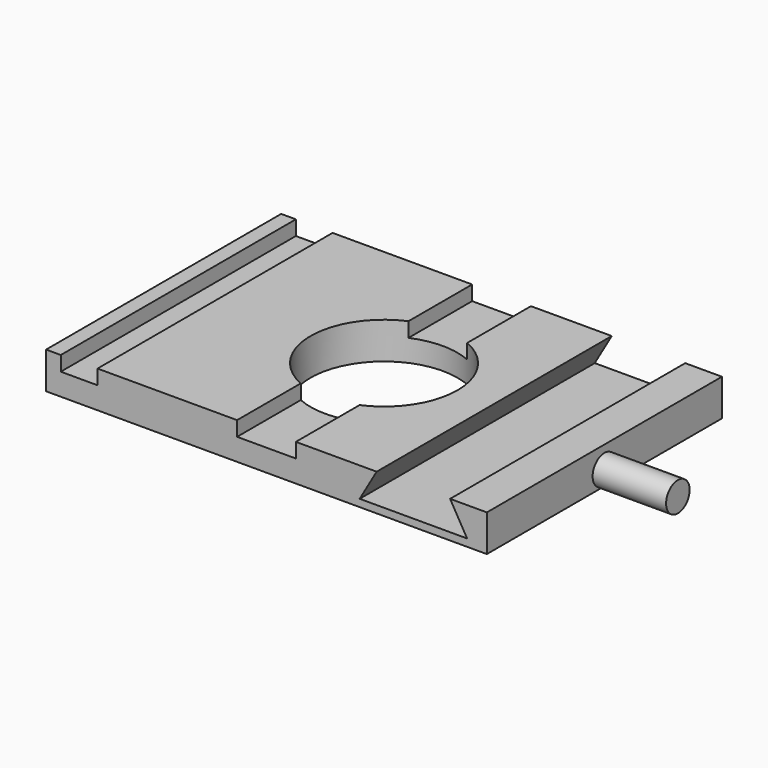
from build123d import *

# Parameters (mm, degrees)
F0_W     = 76.2
F0_H     = 50.8
F0_R     = 12.7
F1_DEPTH = 6.35
F2_W     = 6.35
F2_H     = 50.8
F3_DEPTH = 2.54
F5_DEPTH = 25.4
F6_R     = 2.54
F7_DEPTH = 12.7


# Not quite as in the source:
# - a feature names something its author has since deleted; it is built from what else it names


with BuildPart() as f1:
    # F0 (on Top) → F1 (new body)
    with BuildSketch(Plane.XY):
        Rectangle(F0_W, F0_H)
        Circle(F0_R, mode=Mode.SUBTRACT)
    extrude(amount=-F1_DEPTH)

    # F2 (on face) → F3 (cut)
    with BuildSketch(Plane.XY):
        with Locations((-32.385, 0)):
            Rectangle(F2_W, F2_H)
        with BuildLine():
            Line((-5.08, -11.6397422652), (-5.08, -25.4))
            Line((-5.08, -25.4), (5.08, -25.4))
            Line((5.08, -25.4), (5.08, -11.6397422652))
            ThreePointArc((5.08, -11.6397422652), (0, -12.7), (-5.08, -11.6397422652))
        make_face()
        with BuildLine():
            Line((5.08, 25.4), (-5.08, 25.4))
            Line((-5.08, 25.4), (-5.08, 11.6397422652))
            ThreePointArc((-5.08, 11.6397422652), (0, 12.7), (5.08, 11.6397422652))
            Line((5.08, 11.6397422652), (5.08, 25.4))
        make_face()
    extrude(amount=-F3_DEPTH, mode=Mode.SUBTRACT)

    # F4 (on Front) → F5 (cut, symmetric)
    with BuildSketch(Plane.XZ):
        Polygon((31.75, 0), (19.05, 0), (16.1170606325, -5.08), (34.6859807152, -5.08), align=None)
    extrude(amount=F5_DEPTH, both=True, mode=Mode.SUBTRACT)

    # F6 (on face) → F7 (join)
    with BuildSketch(Plane.YZ.offset(38.1)):
        with Locations((0, -3.81)):
            Circle(F6_R)
    extrude(amount=F7_DEPTH)


solid = f1.part
